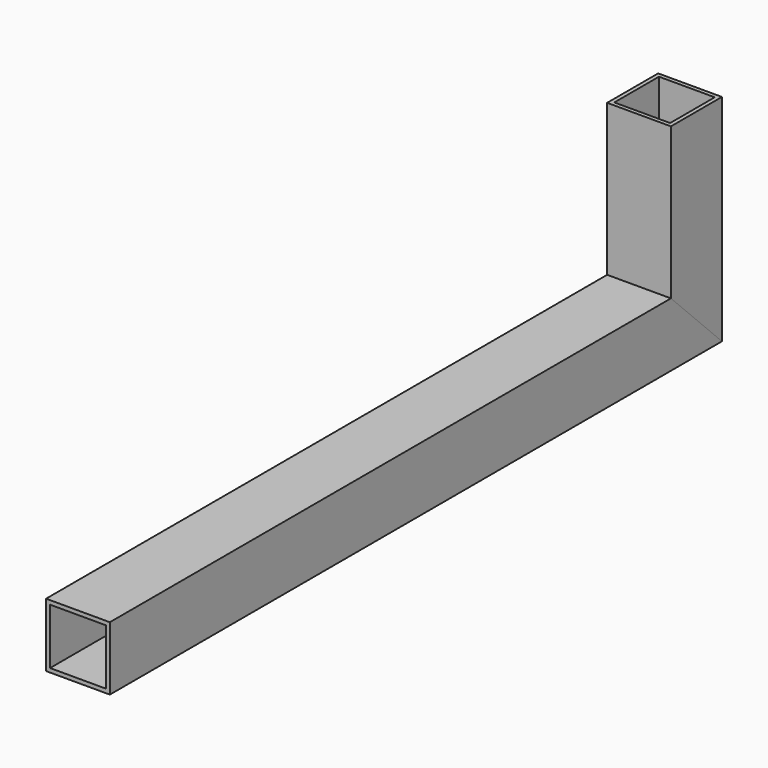
from build123d import *

# Parameters (mm, degrees)
F0_W          = 25.4
F0_H          = 25.4
F0_W_2        = 22.225
F0_H_2        = 22.225
F1_DEPTH      = 304.8
F3_DEPTH      = 12.701
F3_DEPTH_BACK = 12.701
F5_W          = 25.4
F5_H          = 25.4
F5_W_2        = 22.225
F5_H_2        = 22.225
F6_DEPTH      = 60.325
F6_DEPTH_BACK = 50.8
F8_DEPTH      = 25.401


with BuildPart() as f1:
    # F0 (on Front) → F1 (new body)
    with BuildSketch(Plane.XZ):
        Rectangle(F0_W, F0_H)
        Rectangle(F0_W_2, F0_H_2, mode=Mode.SUBTRACT)
    extrude(amount=F1_DEPTH)

    # F2 (on Right) → F3 (cut, two sides)
    with BuildSketch(Plane.YZ) as f3_sk:
        Polygon((0, -12.7), (0, 12.7), (-25.4, 12.7), align=None)
    extrude(amount=-F3_DEPTH, mode=Mode.SUBTRACT)
    extrude(f3_sk.sketch, amount=F3_DEPTH_BACK, mode=Mode.SUBTRACT)


with BuildPart() as f6:
    # F5 (on offset) → F6 (new body, two sides)
    with BuildSketch(Plane.XY.offset(12.7)) as f6_sk:
        with Locations((0, -12.7)):
            Rectangle(F5_W, F5_H)
        with Locations((0, -12.7)):
            Rectangle(F5_W_2, F5_H_2, mode=Mode.SUBTRACT)
    extrude(amount=F6_DEPTH)
    extrude(f6_sk.sketch, amount=-F6_DEPTH_BACK)

    # F7 (on face) → F8 (cut, through all)
    with BuildSketch(Plane.YZ.offset(12.7)):
        Polygon((-25.4, 12.7), (-25.4, -38.1), (0, -38.1), (0, -12.7), align=None)
    extrude(amount=-F8_DEPTH, mode=Mode.SUBTRACT)


solid = Compound([f1.part, f6.part])
